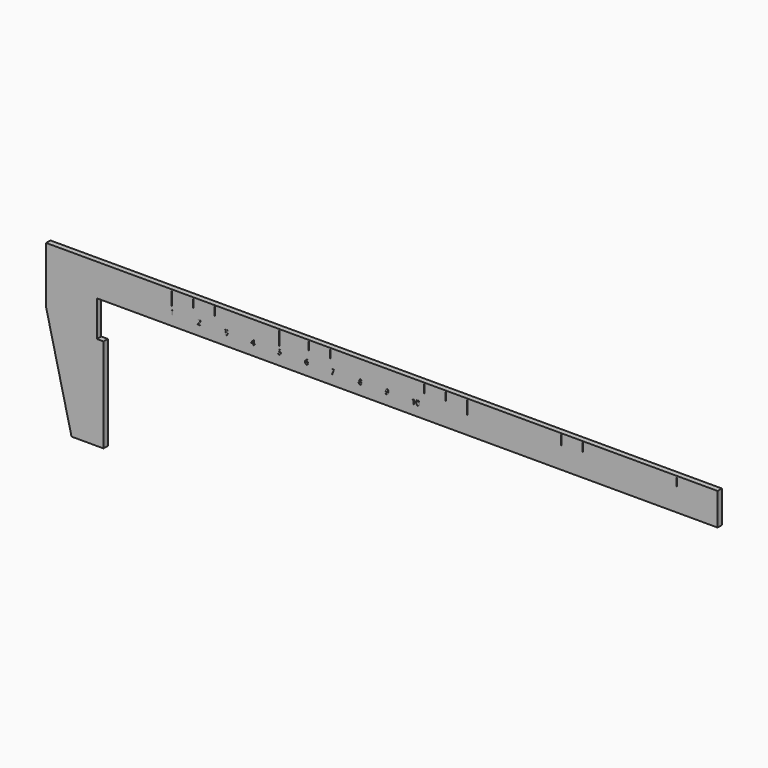
from build123d import *

# Parameters (mm, degrees)
F0_W         = 210
F0_H         = 12
F1_DEPTH     = 2
F2_W         = 0.02
F2_H         = 5
F2_W_2       = 0.01
F2_H_2       = 3
F2_H_3       = 3.5
F2_TEXT_SIZE = 2.6121832586
F3_DEPTH     = 0.1


# Not quite as in the source:
# - Text() gives the source's letters only with a copy of the font that has no kerning and outlines rounded to 1/6400 em; it was checked with that copy


with BuildPart() as f1:
    # F0 (on Front) → F1 (new body)
    with BuildSketch(Plane.XZ):
        with Locations((18.0162531137, 6)):
            Rectangle(F0_W, F0_H)
        Polygon((-86.9837468863, 0), (-86.9837468863, 12), (-126.9837468863, 12), (-126.9837468863, -9.0323425829), (-117.515951395, -48.4097860754), (-105.6048721075, -48.4097860754), (-105.6048721075, -13.3358873427), (-108.0495417442, -13.3305670171), (-108.0495417442, 0), (-105.6048721075, 0), align=None)
    extrude(amount=F1_DEPTH)

    # F2 (on face) → F3 (cut)
    with BuildSketch(Plane.XZ.offset(2)):
        with Locations((-90.1897326112, 9.0057971515)):
            Rectangle(F2_W, F2_H)
        with Locations((-89.1947326112, 10.0057971515)):
            Rectangle(F2_W_2, F2_H_2)
        with Locations((-88.1947326112, 10.0057971515)):
            Rectangle(F2_W_2, F2_H_2)
        with Locations((-87.1947326112, 10.0057971515)):
            Rectangle(F2_W_2, F2_H_2)
        with Locations((-86.1947326112, 10.0057971515)):
            Rectangle(F2_W_2, F2_H_2)
        with Locations((-84.1947326112, 10.0057971515)):
            Rectangle(F2_W_2, F2_H_2)
        with Locations((-83.1947326112, 10.0057971515)):
            Rectangle(F2_W_2, F2_H_2)
        with Locations((-82.1947326112, 10.0057971515)):
            Rectangle(F2_W_2, F2_H_2)
        with Locations((-81.1947326112, 10.0057971515)):
            Rectangle(F2_W_2, F2_H_2)
        with Locations((-85.1947326112, 9.7557971515)):
            Rectangle(F2_W_2, F2_H_3)
        with Locations((-80.1897326112, 9.0057971515)):
            Rectangle(F2_W, F2_H)
        with Locations((-73.1947326112, 10.0057971515)):
            Rectangle(F2_W_2, F2_H_2)
        with Locations((-78.1947326112, 10.0057971515)):
            Rectangle(F2_W_2, F2_H_2)
        with Locations((-76.1947326112, 10.0057971515)):
            Rectangle(F2_W_2, F2_H_2)
        with Locations((-71.1947326112, 10.0057971515)):
            Rectangle(F2_W_2, F2_H_2)
        with Locations((-74.1947326112, 10.0057971515)):
            Rectangle(F2_W_2, F2_H_2)
        with Locations((-75.1947326112, 9.7557971515)):
            Rectangle(F2_W_2, F2_H_3)
        with Locations((-77.1947326112, 10.0057971515)):
            Rectangle(F2_W_2, F2_H_2)
        with Locations((-72.1947326112, 10.0057971515)):
            Rectangle(F2_W_2, F2_H_2)
        with Locations((-79.1947326112, 10.0057971515)):
            Rectangle(F2_W_2, F2_H_2)
        with Locations((-70.1897326112, 9.0057971515)):
            Rectangle(F2_W, F2_H)
        with Locations((-63.1947326112, 10.0057971515)):
            Rectangle(F2_W_2, F2_H_2)
        with Locations((-68.1947326112, 10.0057971515)):
            Rectangle(F2_W_2, F2_H_2)
        with Locations((-66.1947326112, 10.0057971515)):
            Rectangle(F2_W_2, F2_H_2)
        with Locations((-61.1947326112, 10.0057971515)):
            Rectangle(F2_W_2, F2_H_2)
        with Locations((-64.1947326112, 10.0057971515)):
            Rectangle(F2_W_2, F2_H_2)
        with Locations((-65.1947326112, 9.7557971515)):
            Rectangle(F2_W_2, F2_H_3)
        with Locations((-67.1947326112, 10.0057971515)):
            Rectangle(F2_W_2, F2_H_2)
        with Locations((-62.1947326112, 10.0057971515)):
            Rectangle(F2_W_2, F2_H_2)
        with Locations((-69.1947326112, 10.0057971515)):
            Rectangle(F2_W_2, F2_H_2)
        with Locations((-60.1897326112, 9.0057971515)):
            Rectangle(F2_W, F2_H)
        with Locations((-53.1947326112, 10.0057971515)):
            Rectangle(F2_W_2, F2_H_2)
        with Locations((-58.1947326112, 10.0057971515)):
            Rectangle(F2_W_2, F2_H_2)
        with Locations((-56.1947326112, 10.0057971515)):
            Rectangle(F2_W_2, F2_H_2)
        with Locations((-51.1947326112, 10.0057971515)):
            Rectangle(F2_W_2, F2_H_2)
        with Locations((-54.1947326112, 10.0057971515)):
            Rectangle(F2_W_2, F2_H_2)
        with Locations((-55.1947326112, 9.7557971515)):
            Rectangle(F2_W_2, F2_H_3)
        with Locations((-57.1947326112, 10.0057971515)):
            Rectangle(F2_W_2, F2_H_2)
        with Locations((-52.1947326112, 10.0057971515)):
            Rectangle(F2_W_2, F2_H_2)
        with Locations((-59.1947326112, 10.0057971515)):
            Rectangle(F2_W_2, F2_H_2)
        with Locations((-50.1897326112, 9.0057971515)):
            Rectangle(F2_W, F2_H)
        with Locations((-43.1947326112, 10.0057971515)):
            Rectangle(F2_W_2, F2_H_2)
        with Locations((-48.1947326112, 10.0057971515)):
            Rectangle(F2_W_2, F2_H_2)
        with Locations((-46.1947326112, 10.0057971515)):
            Rectangle(F2_W_2, F2_H_2)
        with Locations((-41.1947326112, 10.0057971515)):
            Rectangle(F2_W_2, F2_H_2)
        with Locations((-44.1947326112, 10.0057971515)):
            Rectangle(F2_W_2, F2_H_2)
        with Locations((-45.1947326112, 9.7557971515)):
            Rectangle(F2_W_2, F2_H_3)
        with Locations((-47.1947326112, 10.0057971515)):
            Rectangle(F2_W_2, F2_H_2)
        with Locations((-42.1947326112, 10.0057971515)):
            Rectangle(F2_W_2, F2_H_2)
        with Locations((-49.1947326112, 10.0057971515)):
            Rectangle(F2_W_2, F2_H_2)
        with Locations((-40.1897326112, 9.0057971515)):
            Rectangle(F2_W, F2_H)
        with Locations((-33.1947326112, 10.0057971515)):
            Rectangle(F2_W_2, F2_H_2)
        with Locations((-38.1947326112, 10.0057971515)):
            Rectangle(F2_W_2, F2_H_2)
        with Locations((-36.1947326112, 10.0057971515)):
            Rectangle(F2_W_2, F2_H_2)
        with Locations((-31.1947326112, 10.0057971515)):
            Rectangle(F2_W_2, F2_H_2)
        with Locations((-34.1947326112, 10.0057971515)):
            Rectangle(F2_W_2, F2_H_2)
        with Locations((-35.1947326112, 9.7557971515)):
            Rectangle(F2_W_2, F2_H_3)
        with Locations((-37.1947326112, 10.0057971515)):
            Rectangle(F2_W_2, F2_H_2)
        with Locations((-32.1947326112, 10.0057971515)):
            Rectangle(F2_W_2, F2_H_2)
        with Locations((-39.1947326112, 10.0057971515)):
            Rectangle(F2_W_2, F2_H_2)
        with Locations((-30.1897326112, 9.0057971515)):
            Rectangle(F2_W, F2_H)
        with Locations((-23.1947326112, 10.0057971515)):
            Rectangle(F2_W_2, F2_H_2)
        with Locations((-28.1947326112, 10.0057971515)):
            Rectangle(F2_W_2, F2_H_2)
        with Locations((-26.1947326112, 10.0057971515)):
            Rectangle(F2_W_2, F2_H_2)
        with Locations((-21.1947326112, 10.0057971515)):
            Rectangle(F2_W_2, F2_H_2)
        with Locations((-24.1947326112, 10.0057971515)):
            Rectangle(F2_W_2, F2_H_2)
        with Locations((-25.1947326112, 9.7557971515)):
            Rectangle(F2_W_2, F2_H_3)
        with Locations((-27.1947326112, 10.0057971515)):
            Rectangle(F2_W_2, F2_H_2)
        with Locations((-22.1947326112, 10.0057971515)):
            Rectangle(F2_W_2, F2_H_2)
        with Locations((-29.1947326112, 10.0057971515)):
            Rectangle(F2_W_2, F2_H_2)
        with Locations((-20.1897326112, 9.0057971515)):
            Rectangle(F2_W, F2_H)
        with Locations((-13.1947326112, 10.0057971515)):
            Rectangle(F2_W_2, F2_H_2)
        with Locations((-18.1947326112, 10.0057971515)):
            Rectangle(F2_W_2, F2_H_2)
        with Locations((-16.1947326112, 10.0057971515)):
            Rectangle(F2_W_2, F2_H_2)
        with Locations((-11.1947326112, 10.0057971515)):
            Rectangle(F2_W_2, F2_H_2)
        with Locations((-14.1947326112, 10.0057971515)):
            Rectangle(F2_W_2, F2_H_2)
        with Locations((-15.1947326112, 9.7557971515)):
            Rectangle(F2_W_2, F2_H_3)
        with Locations((-17.1947326112, 10.0057971515)):
            Rectangle(F2_W_2, F2_H_2)
        with Locations((-12.1947326112, 10.0057971515)):
            Rectangle(F2_W_2, F2_H_2)
        with Locations((-19.1947326112, 10.0057971515)):
            Rectangle(F2_W_2, F2_H_2)
        with Locations((-10.1897326112, 9.0057971515)):
            Rectangle(F2_W, F2_H)
        with Locations((-3.1947326112, 10.0057971515)):
            Rectangle(F2_W_2, F2_H_2)
        with Locations((-8.1947326112, 10.0057971515)):
            Rectangle(F2_W_2, F2_H_2)
        with Locations((-6.1947326112, 10.0057971515)):
            Rectangle(F2_W_2, F2_H_2)
        with Locations((-1.1947326112, 10.0057971515)):
            Rectangle(F2_W_2, F2_H_2)
        with Locations((-4.1947326112, 10.0057971515)):
            Rectangle(F2_W_2, F2_H_2)
        with Locations((-5.1947326112, 9.7557971515)):
            Rectangle(F2_W_2, F2_H_3)
        with Locations((-7.1947326112, 10.0057971515)):
            Rectangle(F2_W_2, F2_H_2)
        with Locations((-2.1947326112, 10.0057971515)):
            Rectangle(F2_W_2, F2_H_2)
        with Locations((-9.1947326112, 10.0057971515)):
            Rectangle(F2_W_2, F2_H_2)
        with Locations((-0.1897326112, 9.0057971515)):
            Rectangle(F2_W, F2_H)
        with Locations((6.8052673888, 10.0057971515)):
            Rectangle(F2_W_2, F2_H_2)
        with Locations((1.8052673888, 10.0057971515)):
            Rectangle(F2_W_2, F2_H_2)
        with Locations((3.8052673888, 10.0057971515)):
            Rectangle(F2_W_2, F2_H_2)
        with Locations((8.8052673888, 10.0057971515)):
            Rectangle(F2_W_2, F2_H_2)
        with Locations((5.8052673888, 10.0057971515)):
            Rectangle(F2_W_2, F2_H_2)
        with Locations((4.8052673888, 9.7557971515)):
            Rectangle(F2_W_2, F2_H_3)
        with Locations((2.8052673888, 10.0057971515)):
            Rectangle(F2_W_2, F2_H_2)
        with Locations((7.8052673888, 10.0057971515)):
            Rectangle(F2_W_2, F2_H_2)
        with Locations((0.8052673888, 10.0057971515)):
            Rectangle(F2_W_2, F2_H_2)
        with Locations((9.8102673888, 9.0057971515)):
            Rectangle(F2_W, F2_H)
        with Locations((16.8052673888, 10.0057971515)):
            Rectangle(F2_W_2, F2_H_2)
        with Locations((11.8052673888, 10.0057971515)):
            Rectangle(F2_W_2, F2_H_2)
        with Locations((13.8052673888, 10.0057971515)):
            Rectangle(F2_W_2, F2_H_2)
        with Locations((18.8052673888, 10.0057971515)):
            Rectangle(F2_W_2, F2_H_2)
        with Locations((15.8052673888, 10.0057971515)):
            Rectangle(F2_W_2, F2_H_2)
        with Locations((14.8052673888, 9.7557971515)):
            Rectangle(F2_W_2, F2_H_3)
        with Locations((12.8052673888, 10.0057971515)):
            Rectangle(F2_W_2, F2_H_2)
        with Locations((17.8052673888, 10.0057971515)):
            Rectangle(F2_W_2, F2_H_2)
        with Locations((10.8052673888, 10.0057971515)):
            Rectangle(F2_W_2, F2_H_2)
        with Locations((19.8102673888, 9.0057971515)):
            Rectangle(F2_W, F2_H)
        with Locations((26.8052673888, 10.0057971515)):
            Rectangle(F2_W_2, F2_H_2)
        with Locations((21.8052673888, 10.0057971515)):
            Rectangle(F2_W_2, F2_H_2)
        with Locations((23.8052673888, 10.0057971515)):
            Rectangle(F2_W_2, F2_H_2)
        with Locations((28.8052673888, 10.0057971515)):
            Rectangle(F2_W_2, F2_H_2)
        with Locations((25.8052673888, 10.0057971515)):
            Rectangle(F2_W_2, F2_H_2)
        with Locations((24.8052673888, 9.7557971515)):
            Rectangle(F2_W_2, F2_H_3)
        with Locations((22.8052673888, 10.0057971515)):
            Rectangle(F2_W_2, F2_H_2)
        with Locations((27.8052673888, 10.0057971515)):
            Rectangle(F2_W_2, F2_H_2)
        with Locations((20.8052673888, 10.0057971515)):
            Rectangle(F2_W_2, F2_H_2)
        with Locations((29.8102673888, 9.0057971515)):
            Rectangle(F2_W, F2_H)
        with Locations((36.8052673888, 10.0057971515)):
            Rectangle(F2_W_2, F2_H_2)
        with Locations((31.8052673888, 10.0057971515)):
            Rectangle(F2_W_2, F2_H_2)
        with Locations((33.8052673888, 10.0057971515)):
            Rectangle(F2_W_2, F2_H_2)
        with Locations((38.8052673888, 10.0057971515)):
            Rectangle(F2_W_2, F2_H_2)
        with Locations((35.8052673888, 10.0057971515)):
            Rectangle(F2_W_2, F2_H_2)
        with Locations((34.8052673888, 9.7557971515)):
            Rectangle(F2_W_2, F2_H_3)
        with Locations((32.8052673888, 10.0057971515)):
            Rectangle(F2_W_2, F2_H_2)
        with Locations((37.8052673888, 10.0057971515)):
            Rectangle(F2_W_2, F2_H_2)
        with Locations((30.8052673888, 10.0057971515)):
            Rectangle(F2_W_2, F2_H_2)
        with Locations((39.8102673888, 9.0057971515)):
            Rectangle(F2_W, F2_H)
        with Locations((46.8052673888, 10.0057971515)):
            Rectangle(F2_W_2, F2_H_2)
        with Locations((41.8052673888, 10.0057971515)):
            Rectangle(F2_W_2, F2_H_2)
        with Locations((43.8052673888, 10.0057971515)):
            Rectangle(F2_W_2, F2_H_2)
        with Locations((48.8052673888, 10.0057971515)):
            Rectangle(F2_W_2, F2_H_2)
        with Locations((45.8052673888, 10.0057971515)):
            Rectangle(F2_W_2, F2_H_2)
        with Locations((44.8052673888, 9.7557971515)):
            Rectangle(F2_W_2, F2_H_3)
        with Locations((42.8052673888, 10.0057971515)):
            Rectangle(F2_W_2, F2_H_2)
        with Locations((47.8052673888, 10.0057971515)):
            Rectangle(F2_W_2, F2_H_2)
        with Locations((40.8052673888, 10.0057971515)):
            Rectangle(F2_W_2, F2_H_2)
        with Locations((49.8102673888, 9.0057971515)):
            Rectangle(F2_W, F2_H)
        with Locations((56.8052673888, 10.0057971515)):
            Rectangle(F2_W_2, F2_H_2)
        with Locations((51.8052673888, 10.0057971515)):
            Rectangle(F2_W_2, F2_H_2)
        with Locations((53.8052673888, 10.0057971515)):
            Rectangle(F2_W_2, F2_H_2)
        with Locations((58.8052673888, 10.0057971515)):
            Rectangle(F2_W_2, F2_H_2)
        with Locations((55.8052673888, 10.0057971515)):
            Rectangle(F2_W_2, F2_H_2)
        with Locations((54.8052673888, 9.7557971515)):
            Rectangle(F2_W_2, F2_H_3)
        with Locations((52.8052673888, 10.0057971515)):
            Rectangle(F2_W_2, F2_H_2)
        with Locations((57.8052673888, 10.0057971515)):
            Rectangle(F2_W_2, F2_H_2)
        with Locations((50.8052673888, 10.0057971515)):
            Rectangle(F2_W_2, F2_H_2)
        with Locations((59.8102673888, 9.0057971515)):
            Rectangle(F2_W, F2_H)
        with Locations((66.8052673888, 10.0057971515)):
            Rectangle(F2_W_2, F2_H_2)
        with Locations((61.8052673888, 10.0057971515)):
            Rectangle(F2_W_2, F2_H_2)
        with Locations((63.8052673888, 10.0057971515)):
            Rectangle(F2_W_2, F2_H_2)
        with Locations((68.8052673888, 10.0057971515)):
            Rectangle(F2_W_2, F2_H_2)
        with Locations((65.8052673888, 10.0057971515)):
            Rectangle(F2_W_2, F2_H_2)
        with Locations((64.8052673888, 9.7557971515)):
            Rectangle(F2_W_2, F2_H_3)
        with Locations((62.8052673888, 10.0057971515)):
            Rectangle(F2_W_2, F2_H_2)
        with Locations((67.8052673888, 10.0057971515)):
            Rectangle(F2_W_2, F2_H_2)
        with Locations((60.8052673888, 10.0057971515)):
            Rectangle(F2_W_2, F2_H_2)
        with Locations((69.8102673888, 9.0057971515)):
            Rectangle(F2_W, F2_H)
        with Locations((76.8052673888, 10.0057971515)):
            Rectangle(F2_W_2, F2_H_2)
        with Locations((71.8052673888, 10.0057971515)):
            Rectangle(F2_W_2, F2_H_2)
        with Locations((73.8052673888, 10.0057971515)):
            Rectangle(F2_W_2, F2_H_2)
        with Locations((78.8052673888, 10.0057971515)):
            Rectangle(F2_W_2, F2_H_2)
        with Locations((75.8052673888, 10.0057971515)):
            Rectangle(F2_W_2, F2_H_2)
        with Locations((74.8052673888, 9.7557971515)):
            Rectangle(F2_W_2, F2_H_3)
        with Locations((72.8052673888, 10.0057971515)):
            Rectangle(F2_W_2, F2_H_2)
        with Locations((77.8052673888, 10.0057971515)):
            Rectangle(F2_W_2, F2_H_2)
        with Locations((70.8052673888, 10.0057971515)):
            Rectangle(F2_W_2, F2_H_2)
        with Locations((79.8102673888, 9.0057971515)):
            Rectangle(F2_W, F2_H)
        with Locations((86.8052673888, 10.0057971515)):
            Rectangle(F2_W_2, F2_H_2)
        with Locations((81.8052673888, 10.0057971515)):
            Rectangle(F2_W_2, F2_H_2)
        with Locations((83.8052673888, 10.0057971515)):
            Rectangle(F2_W_2, F2_H_2)
        with Locations((88.8052673888, 10.0057971515)):
            Rectangle(F2_W_2, F2_H_2)
        with Locations((85.8052673888, 10.0057971515)):
            Rectangle(F2_W_2, F2_H_2)
        with Locations((84.8052673888, 9.7557971515)):
            Rectangle(F2_W_2, F2_H_3)
        with Locations((82.8052673888, 10.0057971515)):
            Rectangle(F2_W_2, F2_H_2)
        with Locations((87.8052673888, 10.0057971515)):
            Rectangle(F2_W_2, F2_H_2)
        with Locations((80.8052673888, 10.0057971515)):
            Rectangle(F2_W_2, F2_H_2)
        with Locations((89.8102673888, 9.0057971515)):
            Rectangle(F2_W, F2_H)
        with Locations((96.8052673888, 10.0057971515)):
            Rectangle(F2_W_2, F2_H_2)
        with Locations((91.8052673888, 10.0057971515)):
            Rectangle(F2_W_2, F2_H_2)
        with Locations((93.8052673888, 10.0057971515)):
            Rectangle(F2_W_2, F2_H_2)
        with Locations((98.8052673888, 10.0057971515)):
            Rectangle(F2_W_2, F2_H_2)
        with Locations((95.8052673888, 10.0057971515)):
            Rectangle(F2_W_2, F2_H_2)
        with Locations((94.8052673888, 9.7557971515)):
            Rectangle(F2_W_2, F2_H_3)
        with Locations((92.8052673888, 10.0057971515)):
            Rectangle(F2_W_2, F2_H_2)
        with Locations((97.8052673888, 10.0057971515)):
            Rectangle(F2_W_2, F2_H_2)
        with Locations((90.8052673888, 10.0057971515)):
            Rectangle(F2_W_2, F2_H_2)
        with Locations((99.8102673888, 9.0057971515)):
            Rectangle(F2_W, F2_H)
        with Locations((106.8052673888, 10.0057971515)):
            Rectangle(F2_W_2, F2_H_2)
        with Locations((101.8052673888, 10.0057971515)):
            Rectangle(F2_W_2, F2_H_2)
        with Locations((103.8052673888, 10.0057971515)):
            Rectangle(F2_W_2, F2_H_2)
        with Locations((108.8052673888, 10.0057971515)):
            Rectangle(F2_W_2, F2_H_2)
        with Locations((105.8052673888, 10.0057971515)):
            Rectangle(F2_W_2, F2_H_2)
        with Locations((104.8052673888, 9.7557971515)):
            Rectangle(F2_W_2, F2_H_3)
        with Locations((102.8052673888, 10.0057971515)):
            Rectangle(F2_W_2, F2_H_2)
        with Locations((107.8052673888, 10.0057971515)):
            Rectangle(F2_W_2, F2_H_2)
        with Locations((100.8052673888, 10.0057971515)):
            Rectangle(F2_W_2, F2_H_2)
        with Locations((-80.800935626, 3.5829115659)):
            Text('1', F2_TEXT_SIZE, font='Open Sans', text_align=(TextAlign.LEFT, TextAlign.BOTTOM))
        with Locations((-70.6620663404, 3.5829115659)):
            Text('2', F2_TEXT_SIZE, font='Open Sans', text_align=(TextAlign.LEFT, TextAlign.BOTTOM))
        with Locations((-60.5457909405, 3.5829115659)):
            Text('3', F2_TEXT_SIZE, font='Open Sans', text_align=(TextAlign.LEFT, TextAlign.BOTTOM))
        with Locations((-50.6859831512, 3.5829115659)):
            Text('4', F2_TEXT_SIZE, font='Open Sans', text_align=(TextAlign.LEFT, TextAlign.BOTTOM))
        with Locations((-40.7406911254, 3.5829115659)):
            Text('5', F2_TEXT_SIZE, font='Open Sans', text_align=(TextAlign.LEFT, TextAlign.BOTTOM))
        with Locations((-30.6814070791, 3.5829115659)):
            Text('6', F2_TEXT_SIZE, font='Open Sans', text_align=(TextAlign.LEFT, TextAlign.BOTTOM))
        with Locations((-20.9289509803, 3.5829115659)):
            Text('7', F2_TEXT_SIZE, font='Open Sans', text_align=(TextAlign.LEFT, TextAlign.BOTTOM))
        with Locations((-10.7346791774, 3.5829115659)):
            Text('8', F2_TEXT_SIZE, font='Open Sans', text_align=(TextAlign.LEFT, TextAlign.BOTTOM))
        with Locations((-0.8066745941, 3.5829115659)):
            Text('9', F2_TEXT_SIZE, font='Open Sans', text_align=(TextAlign.LEFT, TextAlign.BOTTOM))
        with Locations((9.1593675315, 3.5829115659)):
            Text('10', F2_TEXT_SIZE, font='Open Sans', text_align=(TextAlign.LEFT, TextAlign.BOTTOM))
    extrude(amount=-F3_DEPTH, mode=Mode.SUBTRACT)


solid = f1.part
